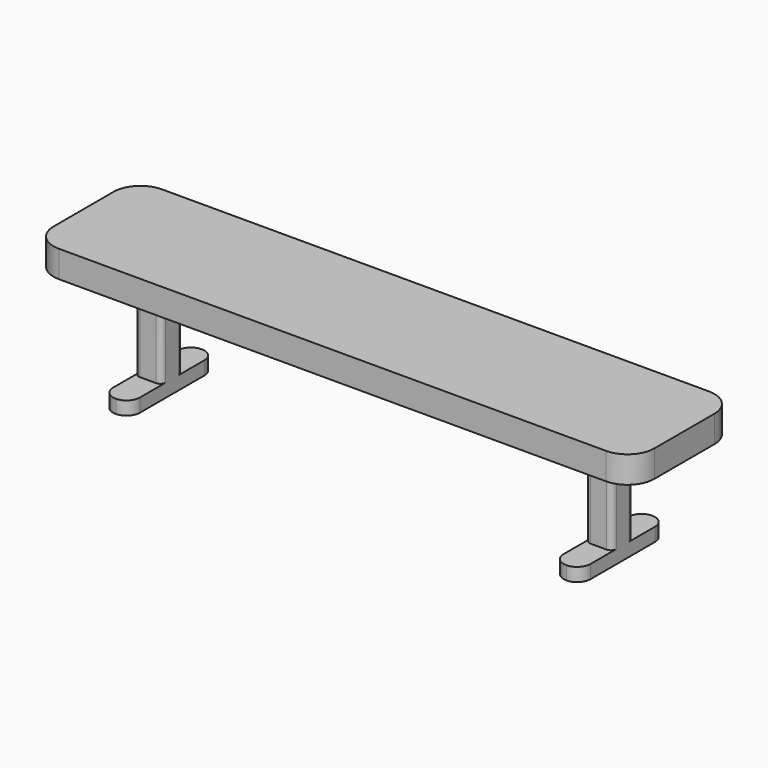
from build123d import *

# Parameters (mm, degrees)
F1_START = 20
F1_DEPTH = 5
F2_DEPTH = 5
F3_R     = 5
F0_W     = 5
F0_H     = 2.5
F4_DEPTH = 25
F0_H_2   = 7.5
F5_DEPTH = 2.5
F6_R     = 1
F7_R     = 2.49999
F8_R     = 2.49999


# Not quite as in the source:
# - a fillet or chamfer is up to 0.001 mm smaller than in the source, because OpenCascade refuses the exact size


with BuildPart() as f1:
    # F0 (on Top) → F1 (new body)
    with BuildSketch(Plane.XY.offset(F1_START)):
        Polygon((56, 0), (56, 12), (-56, 12), (-56, 0), (-44.5, 0), (-44.5, 2.5), (-44.5, 10), (-39.5, 10), (-39.5, 2.5), (-39.5, 0), (-28, 0), (0, 0), (28, 0), (39.5, 0), (39.5, 2.5), (39.5, 10), (44.5, 10), (44.5, 2.5), (44.5, 0), align=None)
        Polygon((56, -12), (56, 0), (44.5, 0), (44.5, -2.5), (44.5, -10), (39.5, -10), (39.5, -2.5), (39.5, 0), (28, 0), (0, 0), (-28, 0), (-39.5, 0), (-39.5, -2.5), (-39.5, -10), (-44.5, -10), (-44.5, -2.5), (-44.5, 0), (-56, 0), (-56, -12), align=None)
    extrude(amount=F1_DEPTH)

    # F2 (add): faces of the model
    f2_faces = [f1.faces().sort_by_distance(p)[0] for p in [
        (39.5, 0, 22.5),
        (-44.5, 0, 22.5),
    ]]
    extrude(f2_faces, amount=F2_DEPTH)

    # F3
    f3_edges = [f1.edges().sort_by_distance(p)[0] for p in [
        (56, -12, 22.5),
        (56, 12, 22.5),
        (-56, -12, 22.5),
        (-56, 12, 22.5),
    ]]
    fillet(f3_edges, radius=F3_R)

    # F0 (on Top) → F4 (join)
    with BuildSketch(Plane.XY):
        with Locations((-42, -1.25)):
            Rectangle(F0_W, F0_H)
        with Locations((-42, 1.25)):
            Rectangle(F0_W, F0_H)
        with Locations((42, 1.25)):
            Rectangle(F0_W, F0_H)
        with Locations((42, -1.25)):
            Rectangle(F0_W, F0_H)
    extrude(amount=F4_DEPTH)

    # F0 (on Top) → F5 (join)
    with BuildSketch(Plane.XY):
        with Locations((-42, -6.25)):
            Rectangle(F0_W, F0_H_2)
        with Locations((-42, 6.25)):
            Rectangle(F0_W, F0_H_2)
        with Locations((42, 6.25)):
            Rectangle(F0_W, F0_H_2)
        with Locations((42, -6.25)):
            Rectangle(F0_W, F0_H_2)
    extrude(amount=F5_DEPTH)

    # F6
    f6_edges = [f1.edges().sort_by_distance(p)[0] for p in [
        (44.5, -2.5, 11.25),
        (39.5, -2.5, 11.25),
        (44.5, 2.5, 11.25),
        (39.5, 2.5, 11.25),
        (-39.5, 2.5, 11.25),
        (-44.5, 2.5, 11.25),
        (-44.5, -2.5, 11.25),
        (-39.5, -2.5, 11.25),
    ]]
    fillet(f6_edges, radius=F6_R)

    # F7 (radius 2.5 in the source; OpenCascade refuses exactly that, so slightly less here)
    f7_edges = [f1.edges().sort_by_distance(p)[0] for p in [
        (-39.5, -10, 1.25),
        (-44.5, -10, 1.25),
        (-39.5, 10, 1.25),
        (-44.5, 10, 1.25),
    ]]
    fillet(f7_edges, radius=F7_R)

    # F8 (radius 2.5 in the source; OpenCascade refuses exactly that, so slightly less here)
    f8_edges = [f1.edges().sort_by_distance(p)[0] for p in [
        (39.5, -10, 1.25),
        (44.5, -10, 1.25),
        (44.5, 10, 1.25),
        (39.5, 10, 1.25),
    ]]
    fillet(f8_edges, radius=F8_R)


solid = f1.part
